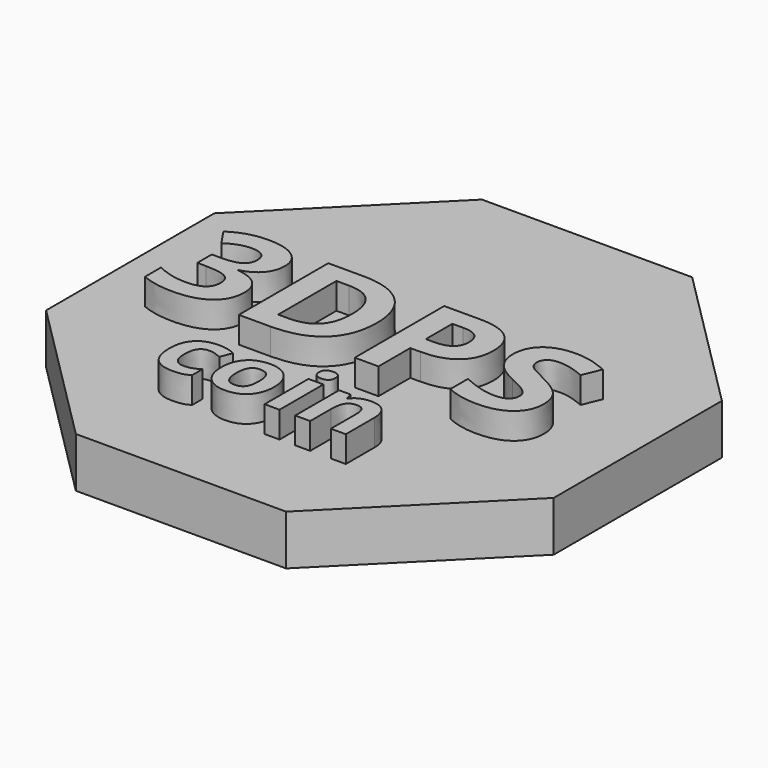
from build123d import *

# Parameters (mm, degrees)
F1_DEPTH     = 3.81
F3_TEXT_SIZE = 11.9276883891
F4_TEXT_SIZE = 7.6462779867
F5_DEPTH     = 2


# Not quite as in the source:
# - Text() gives the source's letters only with a copy of the font that has no kerning and outlines rounded to 1/6400 em; it was checked with that copy


with BuildPart() as f1:
    # F0 (on Top) → F1 (new body)
    with BuildSketch(Plane.XY):
        Polygon((-8.008290664, -19.3337239325), (8.008290664, -19.3337239325), (19.3337239325, -8.008290664), (19.3337239325, 8.008290664), (8.008290664, 19.3337239325), (-8.008290664, 19.3337239325), (-19.3337239325, 8.008290664), (-19.3337239325, -8.008290664), align=None)
    extrude(amount=F1_DEPTH)

    # F3 (on face) + F4 (on face) → F5 (join)
    with BuildSketch(Plane.XY.offset(3.81)):
        with Locations((-15.5019510838, -4.2939676785)):
            Text('3DPS', F3_TEXT_SIZE, font='Open Sans', font_style=FontStyle.BOLD, text_align=(TextAlign.LEFT, TextAlign.BOTTOM))
    with BuildSketch(Plane.XY.offset(3.81)):
        with Locations((-8.4973410703, -12.3271285556)):
            Text('coin', F4_TEXT_SIZE, font='Open Sans', font_style=FontStyle.BOLD, text_align=(TextAlign.LEFT, TextAlign.BOTTOM))
    extrude(amount=F5_DEPTH)


solid = f1.part
